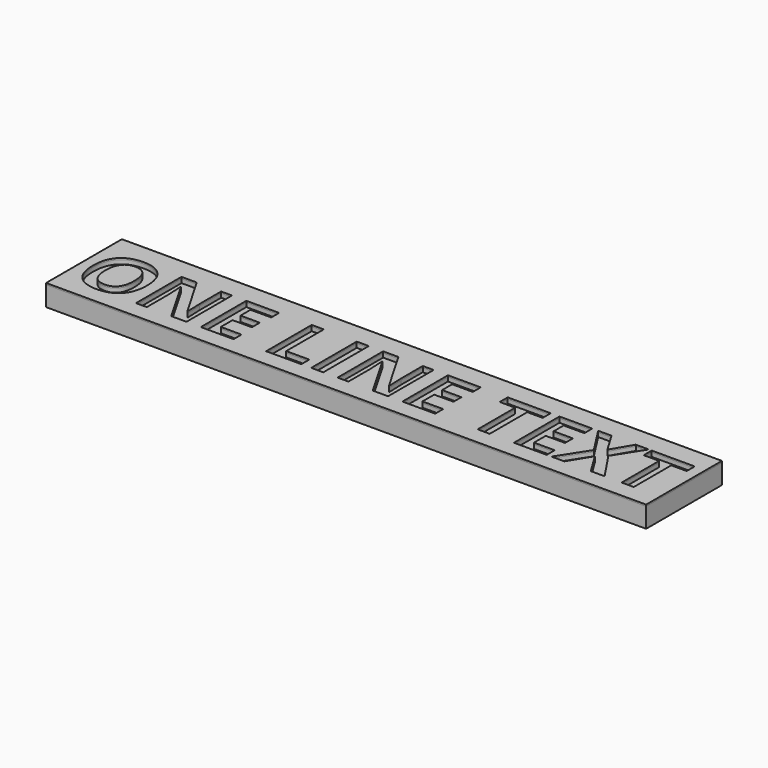
from build123d import *

# Parameters (mm, degrees)
F0_W         = 76
F0_H         = 12
F1_DEPTH     = 2.5
F2_TEXT_SIZE = 10.0979251708
F3_DEPTH     = 0.5
F4_DEPTH     = 0.2


# Not quite as in the source:
# - Text() gives the source's letters only with a copy of the font that has no kerning and outlines rounded to 1/6400 em; it was checked with that copy


with BuildPart() as f1:
    # F0 (on Top) → F1 (new body)
    with BuildSketch(Plane.XY):
        Rectangle(F0_W, F0_H)
    extrude(amount=F1_DEPTH)

    # F2 (on face) → F3 (cut)
    with BuildSketch(Plane.XY.offset(2.5)):
        with Locations((-37.3, -3.8226074957)):
            Text('ONE LINE TEXT', F2_TEXT_SIZE, font='Open Sans', font_style=FontStyle.BOLD, text_align=(TextAlign.LEFT, TextAlign.BOTTOM))
    extrude(amount=-F3_DEPTH, mode=Mode.SUBTRACT)


with BuildPart() as f4:
    # F4 (new): a face of the model
    f4_faces = [f1.part.faces().sort_by_distance(p)[0] for p in [
        (1.1000874922, 0.0497975778, 2.5),
    ]]
    extrude(f4_faces, amount=F4_DEPTH)


with BuildPart() as f4b:
    # F4#2 (new): a face of the model
    f4_2_faces = [f1.part.faces().sort_by_distance(p)[0] for p in [
        (-33.2795549007, -0.2071545508, 2.5),
    ]]
    extrude(f4_2_faces, amount=F4_DEPTH)


solid = Compound([f1.part, f4.part, f4b.part])
